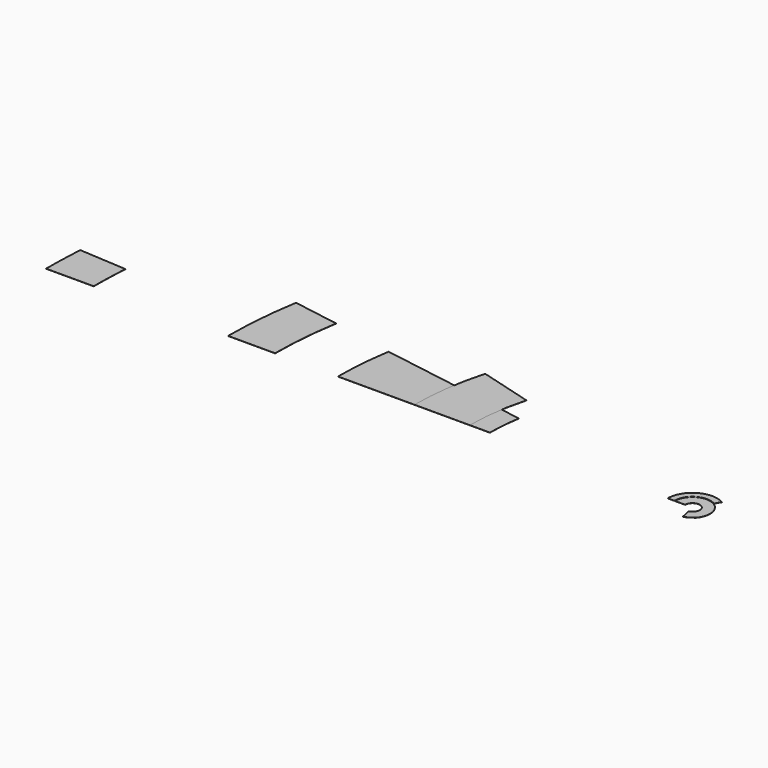
from build123d import *

# Parameters (mm, degrees)
F6_DEPTH = 1
F8_DEPTH = 1


# Not quite as in the source:
# - a feature names something its author has since deleted; it is built from what else it names


with BuildPart() as f6:
    # F0 (on Top) → F6 (new body)
    with BuildSketch(Plane.XY):
        with BuildLine():
            Line((-179, 0), (-131, 0))
            ThreePointArc((-131, 0), (-65.5, 113.4493278958), (65.5, 113.4493278958))
            Line((65.5, 113.4493278958), (89.5, 155.0185472774))
            ThreePointArc((89.5, 155.0185472774), (-89.5, 155.0185472774), (-179, 0))
        make_face()
    extrude(amount=F6_DEPTH)


with BuildPart() as f6b:
    # F2 (on Top) → F6, piece 2 (new body)
    with BuildSketch(Plane.XY):
        with BuildLine():
            Line((-127, 0), (-75, 0))
            ThreePointArc((-75, 0), (29.9061801694, 68.7795055789), (51.1498770047, -54.8515276214))
            Line((51.1498770047, -54.8515276214), (86.6137917279, -92.8819201056))
            ThreePointArc((86.6137917279, -92.8819201056), (50.6411317535, 116.4666294469), (-127, 0))
        make_face()
    extrude(amount=F6_DEPTH)


with BuildPart() as f6c:
    # F4 (on Top) → F6, piece 3 (new body)
    with BuildSketch(Plane.XY):
        with BuildLine():
            Line((-125, 0), (-53, 0))
            ThreePointArc((-53, 0), (32.9932757418, 41.4782323132), (11.9224058802, -51.6416134336))
            Line((11.9224058802, -51.6416134336), (28.118881793, -121.7962580982))
            ThreePointArc((28.118881793, -121.7962580982), (77.8143295797, 97.8260196066), (-125, 0))
        make_face()
    extrude(amount=F6_DEPTH)


with BuildPart() as f6d:
    # F5 (on Top) → F6, piece 4 (new body)
    with BuildSketch(Plane.XY):
        with BuildLine():
            Line((-2567.5, 0), (-1467, 0))
            ThreePointArc((-1467, 0), (-1462.1464470723, 119.2340862083), (-1447.6179041391, 237.6792031622))
            Line((-1447.6179041391, 237.6792031622), (-2533.5780292278, 415.9791098288))
            ThreePointArc((-2533.5780292278, 415.9791098288), (-2559.0054552543, 208.6799702385), (-2567.5, 0))
        make_face()
    extrude(amount=F6_DEPTH)


with BuildPart() as f6e:
    # F3 (on Top) → F6, piece 5 (new body)
    with BuildSketch(Plane.XY):
        with BuildLine():
            Line((-3363.5, 0), (-3023, 0))
            ThreePointArc((-3023, 0), (-3012.5518747764, 251.1179041426), (-2981.2797209521, 500.4999754646))
            Line((-2981.2797209521, 500.4999754646), (-3317.0804966663, 556.8745178548))
            ThreePointArc((-3317.0804966663, 556.8745178548), (-3351.8750350018, 279.4029343644), (-3363.5, 0))
        make_face()
    extrude(amount=F6_DEPTH)


with BuildPart() as f6f:
    # F1 (on Top) → F6, piece 6 (new body)
    with BuildSketch(Plane.XY):
        with BuildLine():
            Line((-4682, 0), (-4337, 0))
            ThreePointArc((-4337, 0), (-4334.80009878, 138.1198885634), (-4328.2026268772, 276.0996571768))
            Line((-4328.2026268772, 276.0996571768), (-4672.5028127828, 298.0628533322))
            ThreePointArc((-4672.5028127828, 298.0628533322), (-4679.6251008734, 149.1070597772), (-4682, 0))
        make_face()
    extrude(amount=F6_DEPTH)


with BuildPart() as f8:
    # F7 (on Top) → F8 (new body)
    with BuildSketch(Plane.XY):
        with BuildLine():
            Line((-2013.34, 0), (-1612.9, 0))
            ThreePointArc((-1612.9, 0), (-1597.718202671, 220.7780669673), (-1552.4586150985, 437.3998838665))
            Line((-1552.4586150985, 437.3998838665), (-1937.8926332212, 545.9945949431))
            ThreePointArc((-1937.8926332212, 545.9945949431), (-1994.3889678006, 275.5913654584), (-2013.34, 0))
        make_face()
    extrude(amount=F8_DEPTH)


solid = Compound([f6.part, f6b.part, f6c.part, f6d.part, f6e.part, f6f.part, f8.part])
